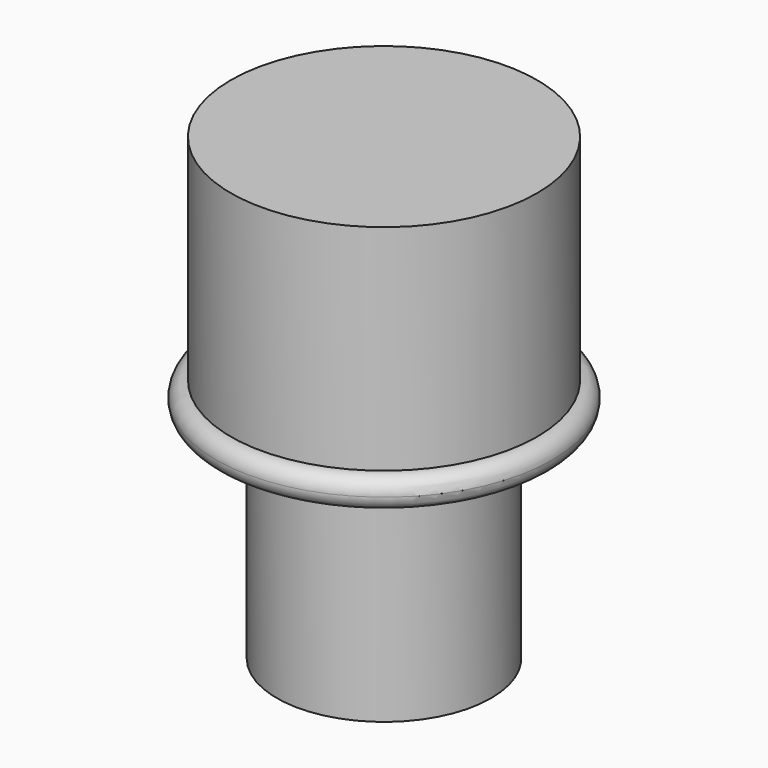
from build123d import *

# Parameters (mm, degrees)
F0_R     = 3.5
F1_DEPTH = 7
F2_R     = 5.5
F3_DEPTH = 1
F5_R     = 0.49999
F4_R     = 5
F6_DEPTH = 7


# Not quite as in the source:
# - a fillet or chamfer is up to 0.001 mm smaller than in the source, because OpenCascade refuses the exact size


with BuildPart() as f1:
    # F0 (on Top) → F1 (new body)
    with BuildSketch(Plane.XY):
        Circle(F0_R)
    extrude(amount=F1_DEPTH)

    # F2 (on face) → F3 (join)
    with BuildSketch(Plane.XY.offset(7)):
        Circle(F2_R)
    extrude(amount=F3_DEPTH)

    # F5 (radius 0.5 in the source; OpenCascade refuses exactly that, so slightly less here)
    f5_edges = [f1.edges().sort_by_distance(p)[0] for p in [
        (-5.5, 0, 8),
        (-5.5, 0, 7),
    ]]
    fillet(f5_edges, radius=F5_R)

    # F4 (on face) → F6 (join)
    with BuildSketch(Plane.XY.offset(8)):
        Circle(F4_R)
    extrude(amount=F6_DEPTH)


solid = f1.part
